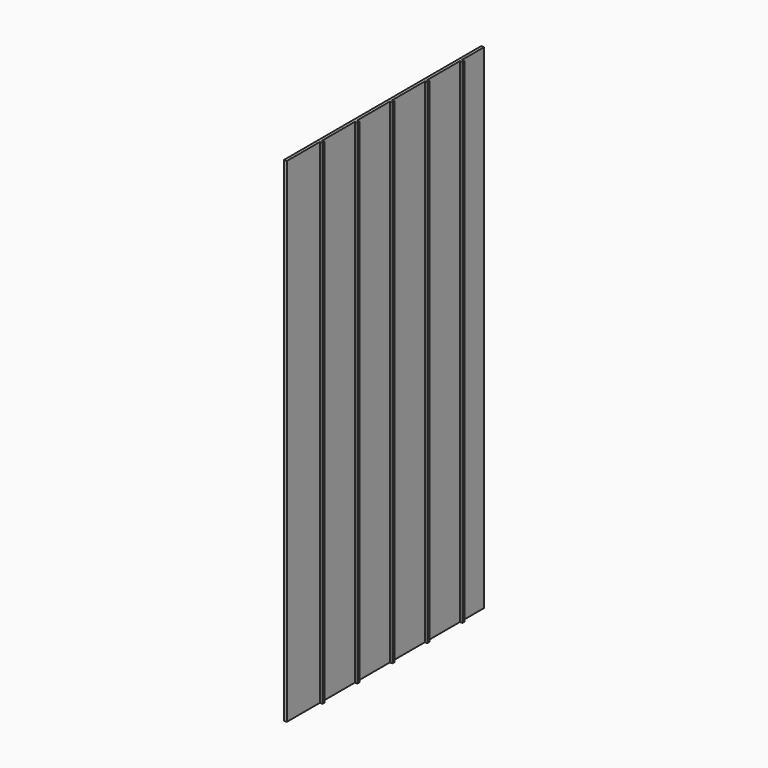
from build123d import *

# Parameters (mm, degrees)
F0_W     = 1215.898
F0_H     = 2435.098
F1_DEPTH = 14.3002
F2_W     = 12.7
F2_H     = 2435.098
F3_DEPTH = 12.7


# Not quite as in the source:
# - a feature names something its author has since deleted; it is built from what else it names


with BuildPart() as f1:
    # F0 (on Right) → F1 (new body)
    with BuildSketch(Plane.YZ):
        with Locations((607.949, 1217.549)):
            Rectangle(F0_W, F0_H)
    extrude(amount=F1_DEPTH)

    # F2 (on face) → F3 (join)
    with BuildSketch(Plane.YZ.offset(14.3002)):
        with Locations((425.45, 1217.549)):
            Rectangle(F2_W, F2_H)
        with Locations((641.35, 1217.549)):
            Rectangle(F2_W, F2_H)
        with Locations((857.25, 1217.549)):
            Rectangle(F2_W, F2_H)
        with Locations((1073.15, 1217.549)):
            Rectangle(F2_W, F2_H)
        with Locations((209.55, 1217.549)):
            Rectangle(F2_W, F2_H)
    extrude(amount=F3_DEPTH)


solid = f1.part
